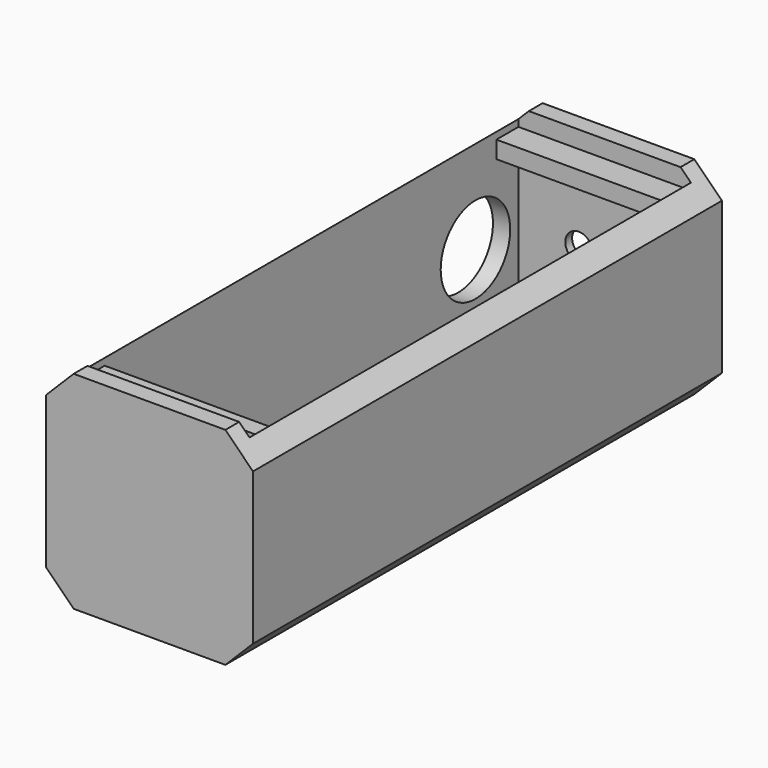
from build123d import *

# Parameters (mm, degrees)
F0_W         = 38.1
F0_H         = 107.95
F1_DEPTH     = 6.35
F2_W         = 22.225
F2_H         = 73.025
F3_DEPTH     = 3.175
F4_W         = 38.1
F4_H         = 107.95
F4_W_2       = 31.75
F4_H_2       = 3.175
F5_DEPTH     = 31.75
F6_R         = 15.875
F6_R_2       = 2.5
F7_DEPTH     = 1.5875
F8_R         = 2.5
F9_DEPTH     = 25.4
F10_R        = 8
F11_DEPTH    = 25.4
F12_W        = 9.525
F12_H        = 3.175
F13_DEPTH    = 25.4
F14_W        = 31.75
F14_H        = 3.175
F15_DEPTH    = 3.175
F16_W        = 5.08
F16_H        = 3.175
F17_DEPTH    = 38.1
F18_T1_DEPTH = 134.0782991577


# Not quite as in the source:
# - a fillet or chamfer that OpenCascade refuses, or shapes differently, is made with other operations: its cross-section is extruded or revolved along the edge and cut away or added


with BuildPart() as f1:
    # F0 (on Top) → F1 (new body)
    with BuildSketch(Plane.XY):
        with Locations((19.05, -53.975)):
            Rectangle(F0_W, F0_H)
    extrude(amount=F1_DEPTH)

    # F2 (on face) → F3 (cut)
    with BuildSketch(Plane.XY.offset(6.35)):
        with Locations((19.05, -61.2775)):
            Rectangle(F2_W, F2_H)
    extrude(amount=-F3_DEPTH, mode=Mode.SUBTRACT)

    # F4 (on face) → F5 (join)
    with BuildSketch(Plane.XY.offset(6.35)):
        with Locations((19.05, -53.975)):
            Rectangle(F4_W, F4_H)
        Polygon((3.175, -98.425), (3.175, -3.175), (34.925, -3.175), (34.925, -98.425), (34.925, -101.6), (34.925, -104.775), (3.175, -104.775), (3.175, -101.6), align=None, mode=Mode.SUBTRACT)
        with Locations((19.05, -100.0125)):
            Rectangle(F4_W_2, F4_H_2)
    extrude(amount=F5_DEPTH)

    # F6 (on face) → F7 (cut)
    with BuildSketch(Plane(origin=(0, 0, 0), x_dir=(-1, 0, 0), z_dir=(0, 1, 0))):
        with Locations((-19.05, 19.05)):
            Circle(F6_R)
        with Locations((-23.8125, 19.05)):
            Circle(F6_R_2, mode=Mode.SUBTRACT)
        with Locations((-14.2875, 19.05)):
            Circle(F6_R_2, mode=Mode.SUBTRACT)
    extrude(amount=-F7_DEPTH, mode=Mode.SUBTRACT)

    # F8 (on face) → F9 (cut)
    with BuildSketch(Plane(origin=(0, 0, 0), x_dir=(-1, 0, 0), z_dir=(0, 1, 0))):
        with Locations((-14.2875, 19.05)):
            Circle(F8_R)
        with Locations((-23.8125, 19.05)):
            Circle(F8_R)
    extrude(amount=-F9_DEPTH, mode=Mode.SUBTRACT)

    # F10 (on face) → F11 (cut)
    with BuildSketch(Plane(origin=(0, 0, 0), x_dir=(0, -1, 0), z_dir=(-1, 0, 0))):
        with Locations((13.08, 19.05)):
            Circle(F10_R)
    extrude(amount=-F11_DEPTH, mode=Mode.SUBTRACT)

    # F12 (on face) → F13 (cut)
    with BuildSketch(Plane.XY.offset(6.35)):
        with Locations((19.05, -103.1875)):
            Rectangle(F12_W, F12_H)
    extrude(amount=-F13_DEPTH, mode=Mode.SUBTRACT)

    # F14 (on face) → F15 (cut)
    with BuildSketch(Plane.XY.offset(38.1)):
        with Locations((19.05, -100.0125)):
            Rectangle(F14_W, F14_H)
    extrude(amount=-F15_DEPTH, mode=Mode.SUBTRACT)

    # F16 (on face) → F17 (join)
    with BuildSketch(Plane.YZ.offset(38.1)):
        with Locations((-5.715, 33.3375)):
            Rectangle(F16_W, F16_H)
    extrude(amount=-F17_DEPTH)

    # F18: chamfer of 5.08 on 4 edges, made by hand

    # F18_s2 → F18_t1 (cut)
    with BuildSketch(Plane.XZ.offset(-13.0641495789)):
        Polygon((38.1, 5.08), (33.02, 0), (38.1, 0), align=None)
        Polygon((38.1, 33.02), (33.02, 38.1), (38.1, 38.1), align=None)
        Polygon((5.08, 38.1), (0, 33.02), (0, 38.1), align=None)
        Polygon((5.08, 0), (0, 5.08), (0, 0), align=None)
    extrude(amount=F18_T1_DEPTH, mode=Mode.SUBTRACT)


solid = f1.part
